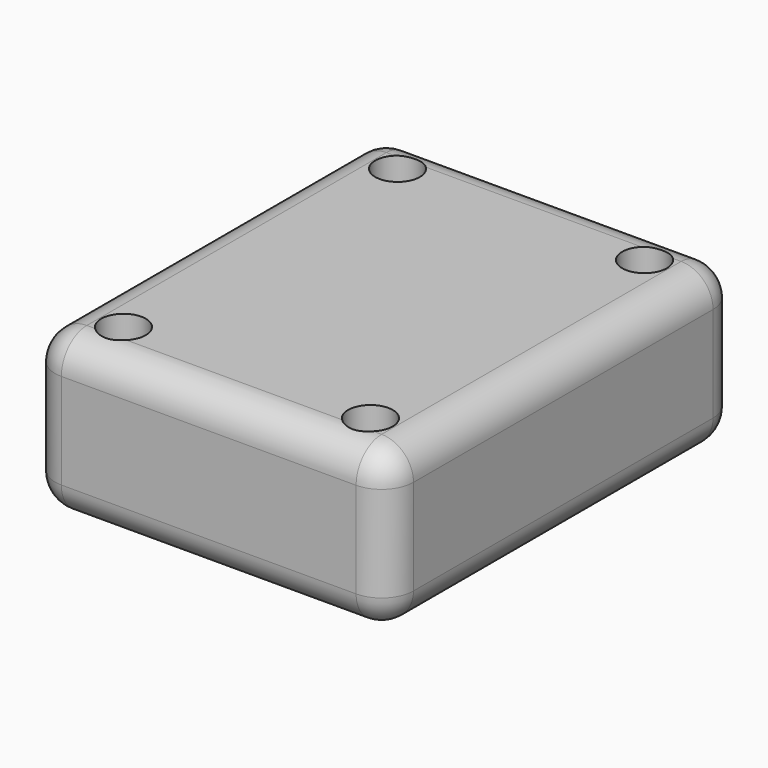
from build123d import *

# Parameters (mm, degrees)
F0_W         = 57.15
F0_H         = 69.85
F1_DEPTH     = 25.4
F2_R         = 3.556
F3_DEPTH     = 25.4
F4_T1_DEPTH  = 82.55
F5_T1_DEPTH  = 77.47
F5_T3_DEPTH  = 33.02
F5_T6_ANGLE  = 89.9999999979
F6_T1_DEPTH  = 64.77
F6_T3_DEPTH  = 33.02
F6_T6_ANGLE  = 89.9999999979
F7_T1_DEPTH  = 59.69
F7_T3_DEPTH  = 33.02
F7_T6_ANGLE  = 89.9999999979
F7_T8_ANGLE  = 89.9999999979
F8_T1_DEPTH  = 59.69
F8_T3_DEPTH  = 46.99
F8_T6_ANGLE  = 89.9999999979
F8_T8_ANGLE  = 90.0000000017
F8_T10_ANGLE = 90.0000000017
F8_T12_ANGLE = 89.9999999979


# Not quite as in the source:
# - a fillet or chamfer that OpenCascade refuses, or shapes differently, is made with other operations: its cross-section is extruded or revolved along the edge and cut away or added


with BuildPart() as f1:
    # F0 (on Top) → F1 (new body)
    with BuildSketch(Plane.XY):
        with Locations((-11.2585859209, 15.0406121326)):
            Rectangle(F0_W, F0_H)
    extrude(amount=F1_DEPTH)

    # F2 (on face) → F3 (cut)
    with BuildSketch(Plane.XY.offset(25.4)):
        with Locations((-30.9435859209, 42.3456121326)):
            Circle(F2_R)
        with Locations((8.4264140791, 42.3456121326)):
            Circle(F2_R)
        with Locations((-30.9435859209, -12.2643878674)):
            Circle(F2_R)
        with Locations((8.4264140791, -12.2643878674)):
            Circle(F2_R)
    extrude(amount=-F3_DEPTH, mode=Mode.SUBTRACT)

    # F4: fillet of radius 5.08 on 1 edges, made by hand

    # F4_s2 → F4_t1 (cut)
    with BuildSketch(Plane.YZ.offset(-52.5335859209)):
        with BuildLine():
            ThreePointArc((-14.8043878674, 25.4), (-18.3964903158, 23.9121024484), (-19.8843878674, 20.32))
            Line((-19.8843878674, 20.32), (-19.8843878674, 25.4))
            Line((-19.8843878674, 25.4), (-14.8043878674, 25.4))
        make_face()
    extrude(amount=F4_T1_DEPTH, mode=Mode.SUBTRACT)

    # F5: fillet of radius 5.08 on 1 edges, made by hand

    # F5_s2 → F5_t1 (cut)
    with BuildSketch(Plane.XZ.offset(-62.6656121326)):
        with BuildLine():
            ThreePointArc((17.3164140791, 20.32), (15.8285165275, 23.9121024484), (12.2364140791, 25.4))
            Line((12.2364140791, 25.4), (17.3164140791, 25.4))
            Line((17.3164140791, 25.4), (17.3164140791, 20.32))
        make_face()
    extrude(amount=F5_T1_DEPTH, mode=Mode.SUBTRACT)

    # F5_s4 → F5_t3 (cut)
    with BuildSketch(Plane.XY.offset(-12.7)):
        with BuildLine():
            ThreePointArc((17.3164140791, -14.8043878674), (15.8285165275, -18.3964903158), (12.2364140791, -19.8843878674))
            Line((12.2364140791, -19.8843878674), (17.3164140791, -19.8843878674))
            Line((17.3164140791, -19.8843878674), (17.3164140791, -14.8043878674))
        make_face()
    extrude(amount=F5_T3_DEPTH, mode=Mode.SUBTRACT)

    # F5_s5 → F5_t6 (revolve, cut)
    with BuildSketch(Plane.XY.offset(20.3199999999)):
        with BuildLine():
            ThreePointArc((17.3164140791, -14.8043878674), (15.8285165275, -18.3964903158), (12.2364140791, -19.8843878674))
            Line((12.2364140791, -19.8843878674), (17.3164140791, -19.8843878674))
            Line((17.3164140791, -19.8843878674), (17.3164140791, -14.8043878674))
        make_face()
    revolve(axis=Axis((17.3164140791, -14.8043878673, 20.3199999999), (-1, 0, 0)), revolution_arc=F5_T6_ANGLE, mode=Mode.SUBTRACT)

    # F6: fillet of radius 5.08 on 1 edges, made by hand

    # F6_s2 → F6_t1 (cut)
    with BuildSketch(Plane.YZ.offset(-52.5335859209)):
        with BuildLine():
            ThreePointArc((49.9656121326, 20.32), (48.477714581, 23.9121024484), (44.8856121326, 25.4))
            Line((44.8856121326, 25.4), (49.9656121326, 25.4))
            Line((49.9656121326, 25.4), (49.9656121326, 20.32))
        make_face()
    extrude(amount=F6_T1_DEPTH, mode=Mode.SUBTRACT)

    # F6_s4 → F6_t3 (cut)
    with BuildSketch(Plane.XY.offset(-12.7)):
        with BuildLine():
            ThreePointArc((12.2364140791, 49.9656121326), (15.8285165275, 48.477714581), (17.3164140791, 44.8856121326))
            Line((17.3164140791, 44.8856121326), (17.3164140791, 49.9656121326))
            Line((17.3164140791, 49.9656121326), (12.2364140791, 49.9656121326))
        make_face()
    extrude(amount=F6_T3_DEPTH, mode=Mode.SUBTRACT)

    # F6_s5 → F6_t6 (revolve, cut)
    with BuildSketch(Plane.YZ.offset(12.236414079)):
        with BuildLine():
            ThreePointArc((49.9656121326, 20.32), (48.477714581, 23.9121024484), (44.8856121326, 25.4))
            Line((44.8856121326, 25.4), (49.9656121326, 25.4))
            Line((49.9656121326, 25.4), (49.9656121326, 20.32))
        make_face()
    revolve(axis=Axis((12.236414079, 49.9656121326, 20.3199999999), (0, 1, 0)), revolution_arc=F6_T6_ANGLE, mode=Mode.SUBTRACT)

    # F7: fillet of radius 5.08 on 1 edges, made by hand

    # F7_s2 → F7_t1 (cut)
    with BuildSketch(Plane.XZ.offset(-44.8856121326)):
        with BuildLine():
            ThreePointArc((-39.8335859209, 20.32), (-38.3456883694, 23.9121024484), (-34.7535859209, 25.4))
            Line((-34.7535859209, 25.4), (-39.8335859209, 25.4))
            Line((-39.8335859209, 25.4), (-39.8335859209, 20.32))
        make_face()
    extrude(amount=F7_T1_DEPTH, mode=Mode.SUBTRACT)

    # F7_s4 → F7_t3 (cut)
    with BuildSketch(Plane.XY.offset(-12.7)):
        with BuildLine():
            ThreePointArc((-39.8335859209, -14.8043878674), (-38.3456883694, -18.3964903158), (-34.7535859209, -19.8843878674))
            Line((-34.7535859209, -19.8843878674), (-39.8335859209, -19.8843878674))
            Line((-39.8335859209, -19.8843878674), (-39.8335859209, -14.8043878674))
        make_face()
        with BuildLine():
            ThreePointArc((-34.7535859209, 49.9656121326), (-38.3456883694, 48.477714581), (-39.8335859209, 44.8856121326))
            Line((-39.8335859209, 44.8856121326), (-39.8335859209, 49.9656121326))
            Line((-39.8335859209, 49.9656121326), (-34.7535859209, 49.9656121326))
        make_face()
    extrude(amount=F7_T3_DEPTH, mode=Mode.SUBTRACT)

    # F7_s5 → F7_t6 (revolve, cut)
    with BuildSketch(Plane.XZ.offset(-44.8856121325)):
        with BuildLine():
            ThreePointArc((-39.8335859209, 20.32), (-38.3456883694, 23.9121024484), (-34.7535859209, 25.4))
            Line((-34.7535859209, 25.4), (-39.8335859209, 25.4))
            Line((-39.8335859209, 25.4), (-39.8335859209, 20.32))
        make_face()
    revolve(axis=Axis((-39.8335859209, 44.8856121325, 20.3199999999), (-1, 0, 0)), revolution_arc=F7_T6_ANGLE, mode=Mode.SUBTRACT)

    # F7_s7 → F7_t8 (revolve, cut)
    with BuildSketch(Plane.XY.offset(20.3199999999)):
        with BuildLine():
            ThreePointArc((-39.8335859209, -14.8043878674), (-38.3456883694, -18.3964903158), (-34.7535859209, -19.8843878674))
            Line((-34.7535859209, -19.8843878674), (-39.8335859209, -19.8843878674))
            Line((-39.8335859209, -19.8843878674), (-39.8335859209, -14.8043878674))
        make_face()
    revolve(axis=Axis((-39.8335859209, -14.8043878673, 20.3199999999), (-1, 0, 0)), revolution_arc=F7_T8_ANGLE, mode=Mode.SUBTRACT)

    # F8: fillet of radius 5.08 on 8 edges, made by hand

    # F8_s2 → F8_t1 (cut)
    with BuildSketch(Plane.XZ.offset(-44.8856121326)):
        with BuildLine():
            ThreePointArc((-34.7535859209, 0), (-38.3456883694, 1.4878975516), (-39.8335859209, 5.08))
            Line((-39.8335859209, 5.08), (-39.8335859209, 0))
            Line((-39.8335859209, 0), (-34.7535859209, 0))
        make_face()
        with BuildLine():
            ThreePointArc((12.2364140791, 0), (15.8285165275, 1.4878975516), (17.3164140791, 5.08))
            Line((17.3164140791, 5.08), (17.3164140791, 0))
            Line((17.3164140791, 0), (12.2364140791, 0))
        make_face()
    extrude(amount=F8_T1_DEPTH, mode=Mode.SUBTRACT)

    # F8_s4 → F8_t3 (cut)
    with BuildSketch(Plane.YZ.offset(-34.7535859209)):
        with BuildLine():
            ThreePointArc((49.9656121326, 5.08), (48.477714581, 1.4878975516), (44.8856121326, 0))
            Line((44.8856121326, 0), (49.9656121326, 0))
            Line((49.9656121326, 0), (49.9656121326, 5.08))
        make_face()
        with BuildLine():
            ThreePointArc((-14.8043878674, 0), (-18.3964903158, 1.4878975516), (-19.8843878674, 5.08))
            Line((-19.8843878674, 5.08), (-19.8843878674, 0))
            Line((-19.8843878674, 0), (-14.8043878674, 0))
        make_face()
    extrude(amount=F8_T3_DEPTH, mode=Mode.SUBTRACT)

    # F8_s5 → F8_t6 (revolve, cut)
    with BuildSketch(Plane.XZ.offset(14.8043878673)):
        with BuildLine():
            ThreePointArc((12.2364140791, 0), (15.8285165275, 1.4878975516), (17.3164140791, 5.08))
            Line((17.3164140791, 5.08), (17.3164140791, 0))
            Line((17.3164140791, 0), (12.2364140791, 0))
        make_face()
    revolve(axis=Axis((12.236414079, -14.8043878673, 0), (0, 0, -1)), revolution_arc=F8_T6_ANGLE, mode=Mode.SUBTRACT)

    # F8_s7 → F8_t8 (revolve, cut)
    with BuildSketch(Plane.YZ.offset(-34.753585921)):
        with BuildLine():
            ThreePointArc((-14.8043878674, 0), (-18.3964903158, 1.4878975516), (-19.8843878674, 5.08))
            Line((-19.8843878674, 5.08), (-19.8843878674, 0))
            Line((-19.8843878674, 0), (-14.8043878674, 0))
        make_face()
    revolve(axis=Axis((-34.753585921, -14.8043878675, 0), (0, 0, -1)), revolution_arc=F8_T8_ANGLE, mode=Mode.SUBTRACT)

    # F8_s9 → F8_t10 (revolve, cut)
    with BuildSketch(Plane.XZ.offset(-44.8856121327)):
        with BuildLine():
            ThreePointArc((-34.7535859209, 0), (-38.3456883693, 1.4878975516), (-39.8335859209, 5.08))
            Line((-39.8335859209, 5.08), (-39.8335859209, 0))
            Line((-39.8335859209, 0), (-34.7535859209, 0))
        make_face()
    revolve(axis=Axis((-34.753585921, 44.8856121327, 0), (0, 0, -1)), revolution_arc=F8_T10_ANGLE, mode=Mode.SUBTRACT)

    # F8_s11 → F8_t12 (revolve, cut)
    with BuildSketch(Plane.YZ.offset(12.236414079)):
        with BuildLine():
            ThreePointArc((44.8856121326, 0), (48.477714581, 1.4878975516), (49.9656121326, 5.08))
            Line((49.9656121326, 5.08), (49.9656121326, 0))
            Line((49.9656121326, 0), (44.8856121326, 0))
        make_face()
    revolve(axis=Axis((12.236414079, 44.8856121325, 0), (0, 0, -1)), revolution_arc=F8_T12_ANGLE, mode=Mode.SUBTRACT)


solid = f1.part
